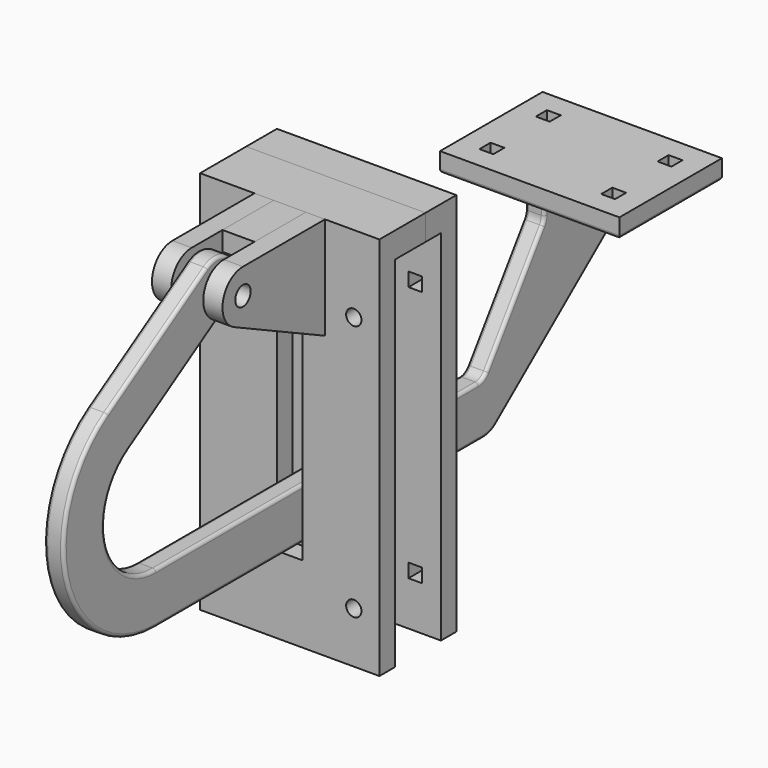
from build123d import *

# Parameters (mm, degrees)
F0_W           = 9.525
F0_H           = 25.4
F0_R           = 4.7752
F1_DEPTH       = 4.7625
F4_R           = 4.7752
F5_DEPTH       = 9.525
F0_H_2         = 44.45
F0_W_2         = 19.05
F0_H_3         = 12.7
F7_DEPTH       = 44.45
F9_W           = 12.7
F9_H           = 139.7
F10_DEPTH      = 76.2
F0_W_3         = 31.75
F0_H_4         = 9.525
F12_DEPTH      = 7.9375
F12_DEPTH_BACK = 7.9375
F13_R          = 1.5875
F14_R          = 1.5875
F15_W          = 6.858
F15_H          = 6.858
F16_DEPTH      = 9.525
F18_D          = 7.62
F19_DEPTH      = 44.45
F21_DEPTH      = 44.45
F21_DEPTH_BACK = 44.45
F22_W          = 12.7
F22_H          = 139.7
F22_W_2        = 6.7564
F22_H_2        = 6.858
F23_DEPTH      = 9.525


# Not quite as in the source:
# - a feature names something its author has since deleted; it is built from what else it names


with BuildPart() as f1:
    # F0 (on Right) → F1 (new body, symmetric)
    with BuildSketch(Plane.YZ):
        with Locations((55.5625, -120.65)):
            Rectangle(F0_W, F0_H)
        with BuildLine():
            Line((-38.1, -133.35), (50.8, -133.35))
            Line((50.8, -133.35), (50.8, -107.95))
            Line((50.8, -107.95), (-38.1, -107.95))
            ThreePointArc((-38.1, -107.95), (-68.6211818995, -84.9475685454), (-54.9180239844, -49.2701546744))
            Line((-54.9180239844, -49.2701546744), (0.8397324108, -14.4487409961))
            Line((0.8397324108, -14.4487409961), (-5.434044736, -11.4787263147))
            ThreePointArc((-5.434044736, -11.4787263147), (-12.6786057506, -0.7368556316), (-6.7272095938, 10.7719381302))
            Line((-6.7272095938, 10.7719381302), (-68.372443172, -27.726278414))
            ThreePointArc((-68.372443172, -27.726278414), (-93.0381274191, -91.9456233818), (-38.1, -133.35))
        make_face()
        with BuildLine():
            Line((60.325, -133.35), (165.1, -133.35))
            ThreePointArc((165.1, -133.35), (167.385363414, -133.1426824208), (169.5961132831, -132.5274982781))
            ThreePointArc((169.5961132831, -132.5274982781), (171.423502452, -131.6637784951), (173.0907217208, -130.521087396))
            Line((173.0907217208, -130.521087396), (257.4506169815, -62.2310986255))
            ThreePointArc((257.4506169815, -62.2310986255), (259.1864445434, -60.0297786323), (259.8052561211, -57.2955549274))
            Line((259.8052561211, -57.2955549274), (259.8052561211, -47.625))
            Line((259.8052561211, -47.625), (202.6552561211, -47.625))
            Line((202.6552561211, -47.625), (202.6552561211, -51.977006656))
            ThreePointArc((202.6552561211, -51.977006656), (202.3624940698, -53.8828839953), (201.5112030715, -55.6130232057))
            Line((201.5112030715, -55.6130232057), (166.8527582665, -105.2360165496))
            ThreePointArc((166.8527582665, -105.2360165496), (164.5822665541, -107.2307728195), (161.646811316, -107.95))
            Line((161.646811316, -107.95), (60.325, -107.95))
            Line((60.325, -107.95), (60.325, -133.35))
        make_face()
        with BuildLine():
            ThreePointArc((0, 12.7), (-3.4990274182, 12.2084727598), (-6.7272095938, 10.7719381302))
            ThreePointArc((-6.7272095938, 10.7719381302), (-12.6786057506, -0.7368556316), (-5.434044736, -11.4787263147))
            Line((-5.434044736, -11.4787263147), (0.8397324108, -14.4487409961))
            Line((0.8397324108, -14.4487409961), (6.7272095938, -10.7719381302))
            ThreePointArc((6.7272095938, -10.7719381302), (12.2084727598, 3.4990274182), (0, 12.7))
        make_face()
        Circle(F0_R, mode=Mode.SUBTRACT)
    extrude(amount=F1_DEPTH, both=True)

    # F13
    f13_edges = [f1.edges().sort_by_distance(p)[0] for p in [
        (4.7625, 164.582267, -107.230773),
        (4.7625, 61.773406, -107.95),
        (4.7625, -68.621182, -84.947569),
        (4.7625, -24.095407, -30.021046),
        (4.7625, -37.549826, -8.47717),
        (4.7625, -93.038127, -91.945623),
        (4.7625, 63.5, -133.35),
        (4.7625, 169.338348, -132.621901),
        (4.7625, 215.270669, -96.376093),
        (4.7625, 10.771938, 6.72721),
        (-4.7625, -37.549826, -8.47717),
        (-4.7625, -93.038127, -91.945623),
        (-4.7625, 10.771938, 6.72721),
        (-4.7625, -24.095407, -30.021046),
        (-4.7625, -68.621182, -84.947569),
        (-4.7625, 61.773406, -107.95),
        (-4.7625, 164.582267, -107.230773),
        (-4.7625, 184.181981, -80.42452),
    ]]
    fillet(f13_edges, radius=F13_R)


with BuildPart() as f5:
    # F4 (on offset) → F5 (new body)
    with BuildSketch(Plane.YZ.offset(7.9375)):
        with BuildLine():
            Line((50.8, 12.7), (0, 12.7))
            ThreePointArc((0, 12.7), (-12.3909205509, 2.7847958456), (-5.434044736, -11.4787263147))
            Line((-5.434044736, -11.4787263147), (50.8, -38.1))
            Line((50.8, -38.1), (50.8, 12.7))
        make_face()
        Circle(F4_R, mode=Mode.SUBTRACT)
    extrude(amount=F5_DEPTH)


with BuildPart() as f6_1:
    # F6: instance of F5
    add(f5.part.mirror(Plane.YZ))


with BuildPart() as f7:
    # F0 (on Right) → F7 (new body, symmetric)
    with BuildSketch(Plane.YZ):
        Polygon((50.8, -107.95), (60.325, -107.95), (60.325, 0), (60.325, 12.7), (50.8, 12.7), (50.8, 3.175), (50.8, -38.1), align=None)
        with Locations((55.5625, -155.575)):
            Rectangle(F0_W, F0_H_2)
        with Locations((55.5625, -120.65)):
            Rectangle(F0_W, F0_H)
        with Locations((69.85, 6.35)):
            Rectangle(F0_W_2, F0_H_3)
    extrude(amount=F7_DEPTH, both=True)


with BuildPart() as f7b:
    # F0 (on Right) → F7, piece 2 (new body, symmetric)
    with BuildSketch(Plane.YZ):
        Polygon((202.6552561211, -47.625), (259.8052561211, -47.625), (262.9802561211, -47.625), (262.9802561211, -38.1), (199.4802561211, -38.1), (199.4802561211, -47.625), align=None)
    extrude(amount=F7_DEPTH, both=True)

    # F14
    f14_edges = [f7b.edges().sort_by_distance(p)[0] for p in [
        (-44.45, 231.230256, -47.625),
        (0, 199.480256, -47.625),
        (44.45, 231.230256, -47.625),
        (0, 262.980256, -47.625),
    ]]
    fillet(f14_edges, radius=F14_R)

    # F15 (on face) → F16 (cut)
    with BuildSketch(Plane(origin=(0, 0, -47.625), x_dir=(1, 0, 0), z_dir=(0, 0, -1))):
        with Locations((-30.1625, -213.7677561211)):
            Rectangle(F15_W, F15_H)
        with Locations((30.1625, -213.7677561211)):
            Rectangle(F15_W, F15_H)
        with Locations((-30.1625, -248.6927561211)):
            Rectangle(F15_W, F15_H)
        with Locations((30.1625, -248.6927561211)):
            Rectangle(F15_W, F15_H)
    extrude(amount=-F16_DEPTH, mode=Mode.SUBTRACT)


with BuildPart() as f10:
    # F9 (on Front) → F10 (new body)
    with BuildSketch(Plane.XZ):
        with Locations((0, -69.85)):
            Rectangle(F9_W, F9_H)
    extrude(amount=-F10_DEPTH)


with BuildPart() as f5_1:
    add(f5.part)

    # F11: cut F10
    add(f10.part, mode=Mode.SUBTRACT)


with BuildPart() as f7_1:
    add(f7.part)

    # F11: cut F10
    add(f10.part, mode=Mode.SUBTRACT)

    # F18 (through all)
    with Locations(Plane.XZ.offset(-50.8)):
        with Locations((31.75, -152.4), (-31.75, -152.4), (31.75, -25.4), (-31.75, -25.4)):
            Hole(F18_D / 2)

    # F0 (on Right) → F19 (join, symmetric)
    with BuildSketch(Plane.YZ):
        with Locations((69.85, 6.35)):
            Rectangle(F0_W_2, F0_H_3)
    extrude(amount=F19_DEPTH, both=True)


with BuildPart() as f12:
    # F0 (on Right) → F12 (new body, two sides)
    with BuildSketch(Plane.YZ) as f12_sk:
        with Locations((34.925, 7.9375)):
            Rectangle(F0_W_3, F0_H_4)
    extrude(amount=F12_DEPTH)
    extrude(f12_sk.sketch, amount=-F12_DEPTH_BACK)


with BuildPart() as f21:
    # F20 (on Right) → F21 (new body, two sides)
    with BuildSketch(Plane.YZ) as f21_sk:
        Polygon((79.375, 0), (88.9, 0), (88.9, -177.8), (98.425, -177.8), (98.425, 12.7), (79.375, 12.7), align=None)
    extrude(amount=F21_DEPTH)
    extrude(f21_sk.sketch, amount=-F21_DEPTH_BACK)

    # F22 (on face) → F23 (cut)
    with BuildSketch(Plane(origin=(0, 98.425, 0), x_dir=(-1, 0, 0), z_dir=(0, 1, 0))):
        with Locations((0, -69.85)):
            Rectangle(F22_W, F22_H)
        with Locations((-31.75, -25.4)):
            Rectangle(F22_W_2, F22_H_2)
        with Locations((31.75, -152.4)):
            Rectangle(F22_W_2, F22_H_2)
        with Locations((-31.75, -152.4)):
            Rectangle(F22_W_2, F22_H_2)
        with Locations((31.75, -25.4)):
            Rectangle(F22_W_2, F22_H_2)
    extrude(amount=-F23_DEPTH, mode=Mode.SUBTRACT)


solid = Compound([f1.part, f6_1.part, f7b.part, f5_1.part, f7_1.part, f12.part, f21.part])
